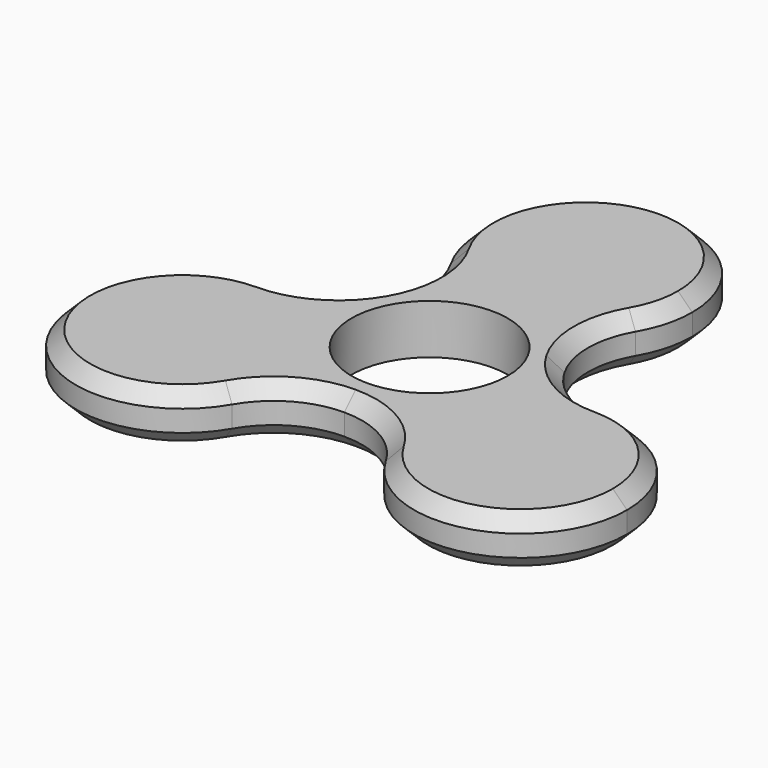
from build123d import *

# Parameters (mm, degrees)
F0_R     = 11
F1_DEPTH = 7
F2_R     = 12.499
F3_SIZE  = 2


# Not quite as in the source:
# - a fillet or chamfer is up to 0.001 mm smaller than in the source, because OpenCascade refuses the exact size


with BuildPart() as f1:
    # F0 (on Top) → F1 (new body)
    with BuildSketch(Plane.XY):
        with BuildLine():
            ThreePointArc((14.9052440041, -1.6833600857), (14.9762922658, -0.8430124372), (15, 0))
            ThreePointArc((15, 0), (12.5483433381, 8.2182163192), (5.9947894041, 13.75))
            ThreePointArc((5.9947894041, 13.75), (0, 12.5), (-5.9947894041, 13.75))
            ThreePointArc((-5.9947894041, 13.75), (-12.9903810568, 7.5), (-14.9052440041, -1.6833600857))
            ThreePointArc((-14.9052440041, -1.6833600857), (-10.8253175473, -6.25), (-8.9104546, -12.0666399143))
            ThreePointArc((-8.9104546, -12.0666399143), (0, -15), (8.9104546, -12.0666399143))
            ThreePointArc((8.9104546, -12.0666399143), (10.8253175473, -6.25), (14.9052440041, -1.6833600857))
        make_face()
        Circle(F0_R, mode=Mode.SUBTRACT)
        with BuildLine():
            ThreePointArc((-5.9947894041, 13.75), (0, 12.5), (5.9947894041, 13.75))
            ThreePointArc((5.9947894041, 13.75), (0, 15), (-5.9947894041, 13.75))
        make_face()
        with BuildLine():
            ThreePointArc((-5.9947894041, 13.75), (0, 15), (5.9947894041, 13.75))
            ThreePointArc((5.9947894041, 13.75), (12.5483433381, 19.2817836808), (15, 27.5))
            ThreePointArc((15, 27.5), (-8.2182163192, 40.0483433381), (-5.9947894041, 13.75))
        make_face()
        with BuildLine():
            ThreePointArc((38.8156986041, -13.75), (30.5737745507, -0.3586442247), (14.9052440041, -1.6833600857))
            ThreePointArc((14.9052440041, -1.6833600857), (12.9903810568, -7.5), (8.9104546, -12.0666399143))
            ThreePointArc((8.9104546, -12.0666399143), (22.9726861669, -28.7262922658), (38.8156986041, -13.75))
        make_face()
        with BuildLine():
            ThreePointArc((8.9104546, -12.0666399143), (12.9903810568, -7.5), (14.9052440041, -1.6833600857))
            ThreePointArc((14.9052440041, -1.6833600857), (10.8253175473, -6.25), (8.9104546, -12.0666399143))
        make_face()
        with BuildLine():
            ThreePointArc((-8.9104546, -12.0666399143), (-10.8253175473, -6.25), (-14.9052440041, -1.6833600857))
            ThreePointArc((-14.9052440041, -1.6833600857), (-12.9903810568, -7.5), (-8.9104546, -12.0666399143))
        make_face()
        with BuildLine():
            ThreePointArc((-8.9104546, -12.0666399143), (-12.9903810568, -7.5), (-14.9052440041, -1.6833600857))
            ThreePointArc((-14.9052440041, -1.6833600857), (-37.2070543793, -20.5080759466), (-8.8156986041, -13.75))
            ThreePointArc((-8.8156986041, -13.75), (-8.8394063383, -12.9069875628), (-8.9104546, -12.0666399143))
        make_face()
    extrude(amount=F1_DEPTH)

    # F2 (radius 12.5 in the source; OpenCascade refuses exactly that, so slightly less here)
    f2_edges = [f1.edges().sort_by_distance(p)[0] for p in [
        (-5.994789, 13.75, 3.5),
        (14.905244, -1.68336, 3.5),
        (-14.905244, -1.68336, 3.5),
        (5.994789, 13.75, 3.5),
        (-8.910455, -12.06664, 3.5),
        (8.910455, -12.06664, 3.5),
    ]]
    fillet(f2_edges, radius=F2_R)

    # F3
    f3_edges = [f1.edges().sort_by_distance(p)[0] for p in [
        (-6.250077, -16.674548, 0),
        (-6.250077, -16.674548, 7),
    ]]
    chamfer(f3_edges, length=F3_SIZE)


solid = f1.part
